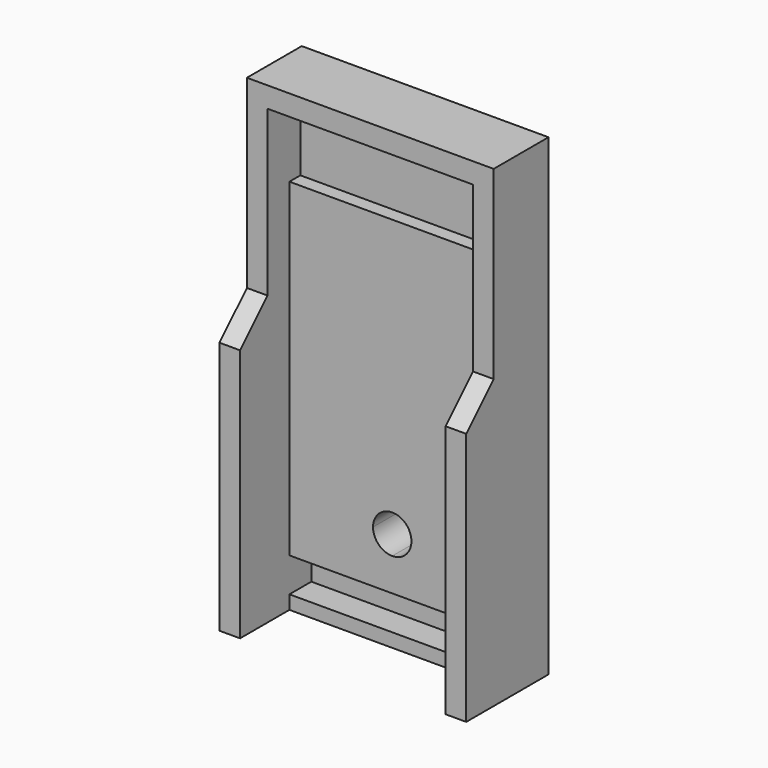
from build123d import *

# Parameters (mm, degrees)
F0_W      = 15
F0_H      = 33
F1_DEPTH  = 3
F2_W      = 15
F2_H      = 2.5
F3_DEPTH  = 2
F4_W      = 15
F4_H      = 5.5
F5_DEPTH  = 1
F7_DEPTH  = 25
F9_DEPTH  = 1.5
F10_W     = 2.5
F10_H     = 21
F11_DEPTH = 1.5
F14_SIZE  = 2.49999
F15_W     = 3
F15_H     = 34.5
F16_DEPTH = 8.25
F17_W     = 8.25
F17_H     = 10
F18_DEPTH = 25
F19_DEPTH = 6
F21_DEPTH = 25
F22_DEPTH = 25


# Not quite as in the source:
# - a fillet or chamfer is up to 0.001 mm smaller than in the source, because OpenCascade refuses the exact size


with BuildPart() as f1:
    # F0 (on Front) → F1 (new body)
    with BuildSketch(Plane.XZ):
        with Locations((7.5, 16.5)):
            Rectangle(F0_W, F0_H)
    extrude(amount=F1_DEPTH)

    # F2 (on face) → F3 (cut)
    with BuildSketch(Plane.XZ.offset(3)):
        with Locations((7.5, 2.25)):
            Rectangle(F2_W, F2_H)
    extrude(amount=-F3_DEPTH, mode=Mode.SUBTRACT)

    # F4 (on face) → F5 (cut)
    with BuildSketch(Plane.XZ.offset(3)):
        with Locations((7.5, 30.25)):
            Rectangle(F4_W, F4_H)
    extrude(amount=-F5_DEPTH, mode=Mode.SUBTRACT)

    # F6 (on face) → F7 (cut)
    with BuildSketch(Plane(origin=(0, 0, 0), x_dir=(-1, 0, 0), z_dir=(0, 1, 0))):
        with BuildLine():
            ThreePointArc((-7.5, 5.9), (-6.5100505063, 6.3100505063), (-6.1, 7.3))
            ThreePointArc((-6.1, 7.3), (-8.4899494937, 8.2899494937), (-7.5, 5.9))
        make_face()
    extrude(amount=-F7_DEPTH, mode=Mode.SUBTRACT)

    # F8 (on face) → F9 (join)
    with BuildSketch(Plane.XY.offset(33)):
        Polygon((16.5, 0), (0, 0), (-1.5, 0), (-1.5, -5), (15, -5), (16.5, -5), align=None)
    extrude(amount=F9_DEPTH)

    # F10 (on face) → F11 (join, through all)
    with BuildSketch(Plane.YZ.offset(16.5)):
        Polygon((0, 34.5), (-5, 34.5), (-5, 21), (-5, 0), (0, 0), align=None)
        with Locations((-6.25, 10.5)):
            Rectangle(F10_W, F10_H)
    extrude(amount=-F11_DEPTH)

    # F13: F1 across plane


with BuildPart() as f1_1:
    add(f1.part)
    add(f1.part.mirror(Plane.YZ.offset(7.5)))

    # F14 (size 2.5 in the source; OpenCascade refuses exactly that, so slightly less here)
    f14_edges = [f1_1.edges().sort_by_distance(p)[0] for p in [
        (15.75, -7.5, 21),
        (-0.75, -7.5, 21),
    ]]
    chamfer(f14_edges, length=F14_SIZE)

    # F15 (on face) → F16 (join)
    with BuildSketch(Plane.YZ.offset(16.5)):
        with Locations((-1.5, 17.25)):
            Rectangle(F15_W, F15_H)
    extrude(amount=F16_DEPTH)

    # F17 (on face) → F18 (cut)
    with BuildSketch(Plane.XZ.offset(3)):
        with Locations((20.625, 29.5)):
            Rectangle(F17_W, F17_H)
    extrude(amount=-F18_DEPTH, mode=Mode.SUBTRACT)

    # F19 (add): a face of the model
    f19_faces = [f1_1.faces().sort_by_distance(p)[0] for p in [
        (20.625, -3, 12.25),
    ]]
    extrude(f19_faces, amount=F19_DEPTH)

    # F20 (on face) → F21 (cut)
    with BuildSketch(Plane(origin=(0, 0, 0), x_dir=(-1, 0, 0), z_dir=(0, 1, 0))):
        with BuildLine():
            ThreePointArc((-22.15, 8.3), (-20.75, 6.9), (-19.35, 8.3))
            Line((-19.35, 8.3), (-20.75, 8.3))
            Line((-20.75, 8.3), (-22.15, 8.3))
        make_face()
        with BuildLine():
            Line((-20.75, 8.3), (-19.35, 8.3))
            ThreePointArc((-19.35, 8.3), (-19.7600505063, 9.2899494937), (-20.75, 9.7))
            Line((-20.75, 9.7), (-20.75, 8.3))
        make_face()
        with BuildLine():
            ThreePointArc((-19.35, 18.3), (-21.7399494937, 19.2899494937), (-20.75, 16.9))
            ThreePointArc((-20.75, 16.9), (-19.7600505063, 17.3100505063), (-19.35, 18.3))
        make_face()
        with BuildLine():
            Line((-22.15, 8.3), (-20.75, 8.3))
            Line((-20.75, 8.3), (-20.75, 9.7))
            ThreePointArc((-20.75, 9.7), (-21.7399494937, 9.2899494937), (-22.15, 8.3))
        make_face()
    extrude(amount=-F21_DEPTH, mode=Mode.SUBTRACT)

    # F22 (cut): a face of the model
    f22_faces = [f1_1.faces().sort_by_distance(p)[0] for p in [
        (20.625, -4.5, 24.5),
    ]]
    extrude(f22_faces, amount=-F22_DEPTH, mode=Mode.SUBTRACT)


solid = f1_1.part
